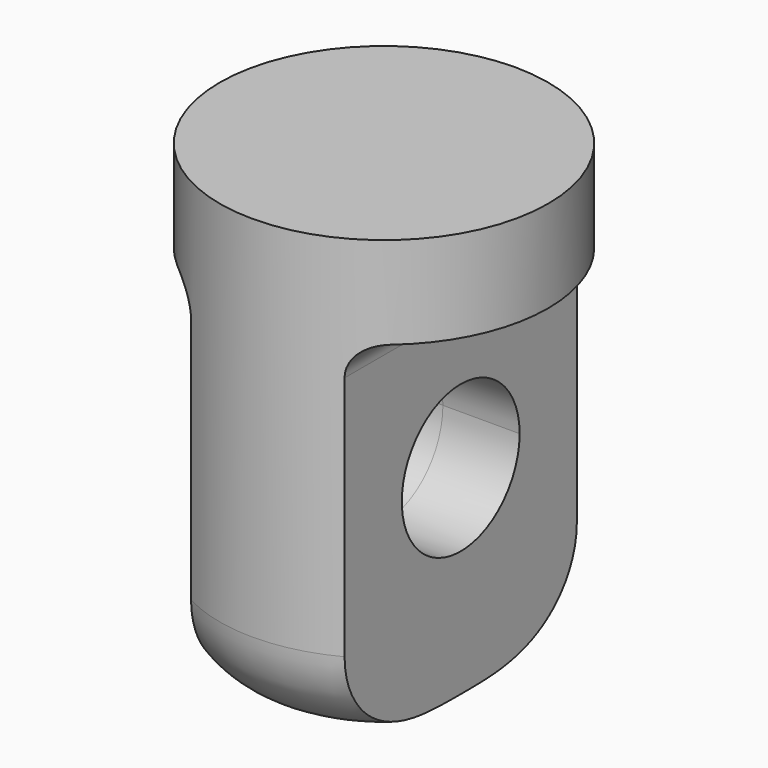
from build123d import *
from build123d import SkipClean  # not in build123d's __all__

# Parameters (mm, degrees)
F0_R     = 10.7
F1_DEPTH = 30
F2_R     = 6
F4_DEPTH = 10.701
F5_DEPTH = 10.7010001
F6_W     = 6.2500013784
F6_H     = 36.9480545221
F6_W_2   = 6.8020046502
F6_H_2   = 40.0000055429
F7_DEPTH = 24
F8_R     = 2


# Not quite as in the source:
# - after a boolean that leaves OpenCascade's solid faulty, fix() repairs it


with BuildPart() as f1:
    # F0 (on Top) → F1 (new body)
    with BuildSketch(Plane.XY):
        Circle(F0_R)
    extrude(amount=-F1_DEPTH)

    # F2
    f2_edges = [f1.edges().sort_by_distance(p)[0] for p in [
        (-10.7, 0, -30),
    ]]
    fillet(f2_edges, radius=F2_R)

    # F3 (on Right) → F4 (cut, through all)
    with BuildSketch(Plane.YZ):
        with BuildLine():
            ThreePointArc((0, -12.2), (-3.3941125497, -20.3941125497), (4.8, -17))
            ThreePointArc((4.8, -17), (3.3941125497, -13.6058874503), (0, -12.2))
        make_face()
    extrude(amount=-F4_DEPTH, mode=Mode.SUBTRACT)

    # F5 (cut, through all): a face of the model
    f5_faces = [f1.faces().sort_by_distance(p)[0] for p in [
        (0, 0, -17),
    ]]
    with SkipClean():  # cleaning this boolean's faces spoils the solid; the shape is the same uncleaned
        extrude(f5_faces, amount=-F5_DEPTH, mode=Mode.SUBTRACT)

    # F6 (on face) → F7 (cut)
    with BuildSketch(Plane(origin=(0, 0, -30), x_dir=(1, 0, 0), z_dir=(0, 0, -1))):
        with Locations((-8.1250006892, 1.5259755104)):
            Rectangle(F6_W, F6_H)
        with Locations((8.4010023251, 0)):
            Rectangle(F6_W_2, F6_H_2)
    extrude(amount=-F7_DEPTH, mode=Mode.SUBTRACT)

    add(f1.part.fix(), mode=Mode.REPLACE)

    # F8
    f8_edges = [f1.edges().sort_by_distance(p)[0] for p in [
        (-5, 0, -6),
        (5, 0, -6),
    ]]
    fillet(f8_edges, radius=F8_R)


solid = f1.part
